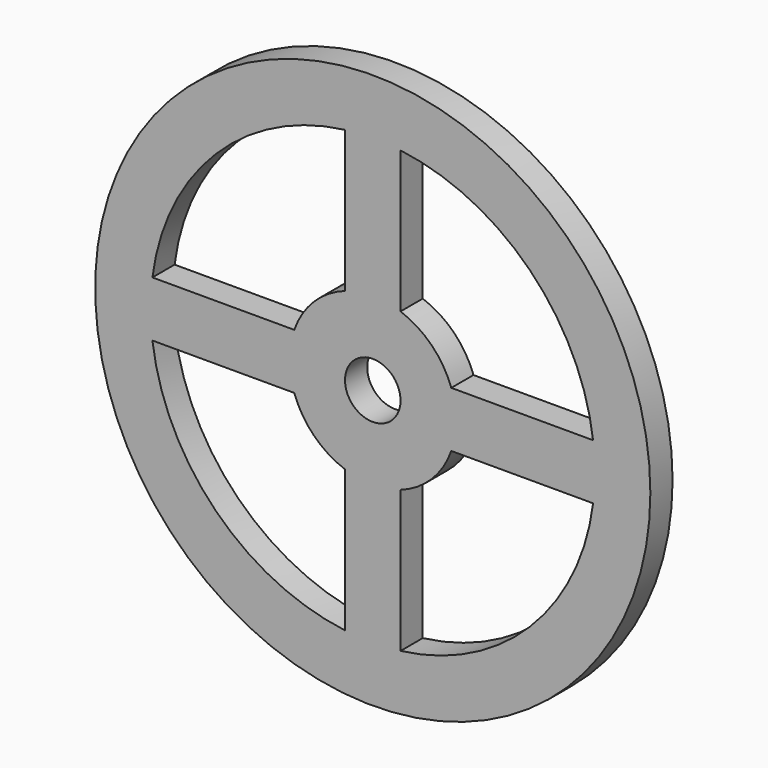
from build123d import *

# Parameters (mm, degrees)
F0_R     = 63.5
F0_R_2   = 6.35
F1_DEPTH = 3.175


# Not quite as in the source:
# - a feature of the source that left no trace in its solid (it failed there, or was rolled back) is left out


with BuildPart() as f1:
    # F0 (on Front) → F1 (new body, symmetric)
    with BuildSketch(Plane.XZ):
        Circle(F0_R)
        with BuildLine():
            ThreePointArc((-6.35, -50.4015624758), (-35.9210244843, -35.9210244843), (-50.4015624758, -6.35))
            Line((-50.4015624758, -6.35), (-17.9605122421, -6.35))
            ThreePointArc((-17.9605122421, -6.35), (-13.4703841816, -13.4703841816), (-6.35, -17.9605122421))
            Line((-6.35, -17.9605122421), (-6.35, -50.4015624758))
        make_face(mode=Mode.SUBTRACT)
        with BuildLine():
            ThreePointArc((50.4015624758, -6.35), (35.9210244843, -35.9210244843), (6.35, -50.4015624758))
            Line((6.35, -50.4015624758), (6.35, -17.9605122421))
            ThreePointArc((6.35, -17.9605122421), (13.4703841816, -13.4703841816), (17.9605122421, -6.35))
            Line((17.9605122421, -6.35), (50.4015624758, -6.35))
        make_face(mode=Mode.SUBTRACT)
        with BuildLine():
            ThreePointArc((-50.4015624758, 6.35), (-35.9210244843, 35.9210244843), (-6.35, 50.4015624758))
            Line((-6.35, 50.4015624758), (-6.35, 17.9605122421))
            ThreePointArc((-6.35, 17.9605122421), (-13.4703841816, 13.4703841816), (-17.9605122421, 6.35))
            Line((-17.9605122421, 6.35), (-50.4015624758, 6.35))
        make_face(mode=Mode.SUBTRACT)
        Circle(F0_R_2, mode=Mode.SUBTRACT)
        with BuildLine():
            Line((50.4015624758, 6.35), (17.9605122421, 6.35))
            ThreePointArc((17.9605122421, 6.35), (13.4703841816, 13.4703841816), (6.35, 17.9605122421))
            Line((6.35, 17.9605122421), (6.35, 50.4015624758))
            ThreePointArc((6.35, 50.4015624758), (35.9210244843, 35.9210244843), (50.4015624758, 6.35))
        make_face(mode=Mode.SUBTRACT)
    extrude(amount=F1_DEPTH, both=True)


solid = f1.part
